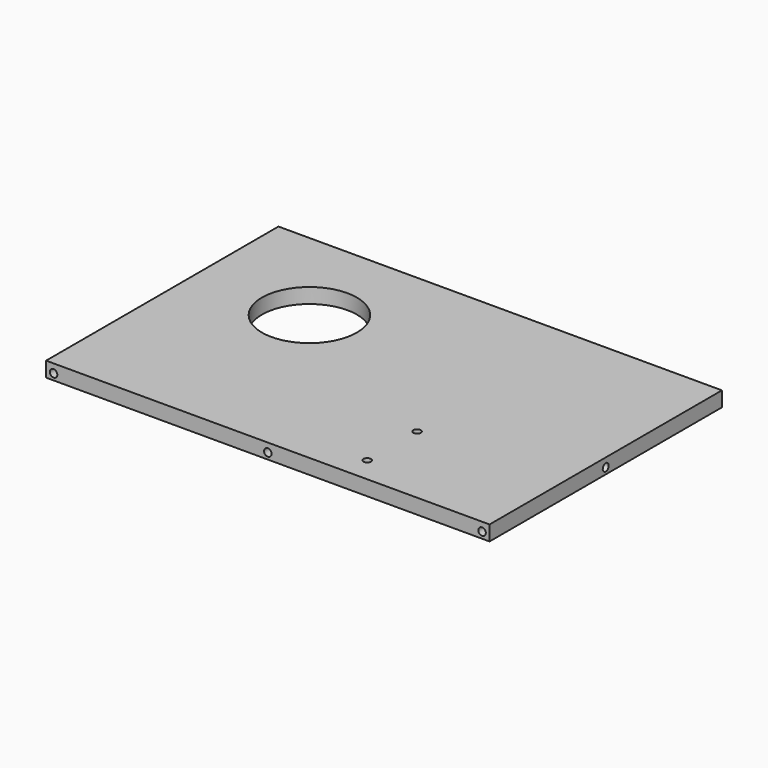
from build123d import *

# Parameters (mm, degrees)
F0_R      = 19
F1_DEPTH  = 6
F2_START  = 3
F0_R_2    = 1.5
F2_DEPTH  = 3
F3_R      = 1.5
F4_DEPTH  = 8
F5_R      = 1.5
F6_DEPTH  = 8
F7_R      = 1.5
F8_DEPTH  = 5
F9_R      = 1.5
F10_DEPTH = 5


# Not quite as in the source:
# - a feature names something its author has since deleted; it is built from what else it names


with BuildPart() as f1:
    # F0 (on Top) → F1 (new body)
    with BuildSketch(Plane.XY):
        Polygon((0, 116.25), (0, 0), (177.5, 0), (177.5, 5), (177.5, 40), (177.5, 52.125), (177.5, 64.125), (177.5, 116.25), align=None)
        with BuildLine():
            ThreePointArc((123, 40), (126, 37), (123, 34))
            Line((123, 34), (123, 11))
            ThreePointArc((123, 11), (126, 8), (123, 5))
            Line((123, 5), (118, 5))
            ThreePointArc((118, 5), (115, 8), (118, 11))
            Line((118, 11), (118, 34))
            ThreePointArc((118, 34), (115, 37), (118, 40))
            Line((118, 40), (123, 40))
        make_face(mode=Mode.SUBTRACT)
        with Locations((45, 75.5)):
            Circle(F0_R, mode=Mode.SUBTRACT)
    extrude(amount=F1_DEPTH)

    # F0 (on Top) → F2 (join)
    with BuildSketch(Plane.XY.offset(F2_START)):
        with BuildLine():
            Line((123, 11), (123, 34))
            ThreePointArc((123, 34), (126, 37), (123, 40))
            Line((123, 40), (118, 40))
            ThreePointArc((118, 40), (115, 37), (118, 34))
            Line((118, 34), (118, 11))
            ThreePointArc((118, 11), (115, 8), (118, 5))
            Line((118, 5), (123, 5))
            ThreePointArc((123, 5), (126, 8), (123, 11))
        make_face()
        with Locations((120.5, 10)):
            Circle(F0_R_2, mode=Mode.SUBTRACT)
        with Locations((120.5, 35)):
            Circle(F0_R_2, mode=Mode.SUBTRACT)
    extrude(amount=F2_DEPTH)

    # F3 (on face) → F4 (cut)
    with BuildSketch(Plane.YZ.offset(177.5)):
        with Locations((58.125, 2.5)):
            Circle(F3_R)
    extrude(amount=-F4_DEPTH, mode=Mode.SUBTRACT)

    # F5 (on face) → F6 (cut)
    with BuildSketch(Plane(origin=(0, 0, 0), x_dir=(0, -1, 0), z_dir=(-1, 0, 0))):
        with Locations((-58.125, 2.5)):
            Circle(F5_R)
    extrude(amount=-F6_DEPTH, mode=Mode.SUBTRACT)

    # F7 (on face) → F8 (cut)
    with BuildSketch(Plane.XZ):
        with Locations((3, 2.5)):
            Circle(F7_R)
        with Locations((88.75, 2.5)):
            Circle(F7_R)
        with Locations((174.5, 2.5)):
            Circle(F7_R)
    extrude(amount=-F8_DEPTH, mode=Mode.SUBTRACT)

    # F9 (on face) → F10 (cut)
    with BuildSketch(Plane(origin=(0, 116.25, 0), x_dir=(-1, 0, 0), z_dir=(0, 1, 0))):
        with Locations((-3, 2.5)):
            Circle(F9_R)
        with Locations((-88.75, 2.5)):
            Circle(F9_R)
        with Locations((-174.5, 2.5)):
            Circle(F9_R)
    extrude(amount=-F10_DEPTH, mode=Mode.SUBTRACT)


solid = f1.part
